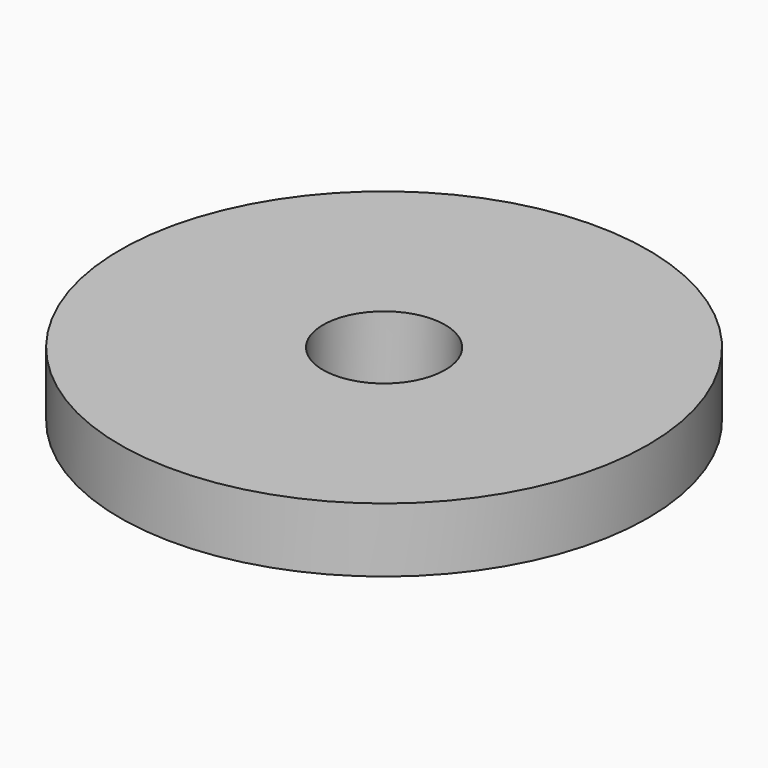
from build123d import *

# Parameters (mm, degrees)
F0_R            = 34.0451530949
F0_R_2          = 1.25
F0_R_3          = 7.875
F1_DEPTH        = 4.15
F3_DEPTH        = 1.25
F3_COPIES_COUNT = 4


# Not quite as in the source:
# - a pattern or mirror of a feature is missing from the dataset's text; its kind, count and spacing are read off the source's solid


with BuildPart() as f1:
    # F0 (on Top) → F1 (new body, symmetric)
    with BuildSketch(Plane.XY):
        Circle(F0_R)
        with Locations((10.6066017178, -10.6066017178)):
            Circle(F0_R_2, mode=Mode.SUBTRACT)
        Circle(F0_R_3, mode=Mode.SUBTRACT)
        with Locations((15, 0)):
            Circle(F0_R_2, mode=Mode.SUBTRACT)
        with Locations((10.6066017178, 10.6066017178)):
            Circle(F0_R_2, mode=Mode.SUBTRACT)
        with Locations((10.6066017178, 10.6066017178)):
            Circle(F0_R_2)
        with Locations((15, 0)):
            Circle(F0_R_2)
        with Locations((10.6066017178, -10.6066017178)):
            Circle(F0_R_2)
    extrude(amount=F1_DEPTH, both=True)

    # F2 (on Top) → F3 (cut, symmetric)
    with BuildSketch(Plane.XY):
        with BuildLine():
            Line((9.4432745967, 10.1492506389), (13.2777855897, 0.3957137164))
            ThreePointArc((13.2777855897, 0.3957137164), (13.3159783656, 0.3022787926), (13.3566720831, 0.2099056662))
            Line((13.3566720831, 0.2099056662), (6.3440025672, -6.039136155))
            ThreePointArc((6.3440025672, -6.039136155), (6.6944330225, -11.915202943), (12.3288161281, -10.2108880014))
            Line((12.3288161281, -10.2108880014), (15.6329589882, -1.8064058021))
            ThreePointArc((15.6329589882, -1.8064058021), (20.0264439119, -0.0879066383), (19.2625991506, 4.5674655628))
            Line((19.2625991506, 4.5674655628), (11.4382124503, 11.5398345877))
            ThreePointArc((11.4382124503, 11.5398345877), (9.891801137, 11.6320577772), (9.4432745967, 10.1492506389))
        make_face()
        with BuildLine():
            ThreePointArc((10.0021618859, -9.2961858437), (8.1240341841, -9.8642908242), (8.0072240323, -7.9056018949))
            Line((8.0072240323, -7.9056018949), (11.9194173824, -4.4194173824))
            Line((11.9194173824, -4.4194173824), (10.0021618859, -9.2961858437))
        make_face(mode=Mode.SUBTRACT)
        with BuildLine():
            ThreePointArc((17.5993776855, 2.7009998229), (17.4825675337, 0.7423108936), (15.6044398319, 1.3104158741))
            Line((15.6044398319, 1.3104158741), (13.6871843354, 6.1871843354))
            Line((13.6871843354, 6.1871843354), (17.5993776855, 2.7009998229))
        make_face(mode=Mode.SUBTRACT)
    f3 = extrude(amount=F3_DEPTH, both=True, mode=Mode.SUBTRACT)

    # F3_copies: F3 ×4 about axis
    f3_copies_axis = Axis((0, 0, 0), (0, 0, 1))
    for i in range(1, F3_COPIES_COUNT):
        add(f3.rotate(f3_copies_axis, i * 360 / F3_COPIES_COUNT), mode=Mode.SUBTRACT)


solid = f1.part
